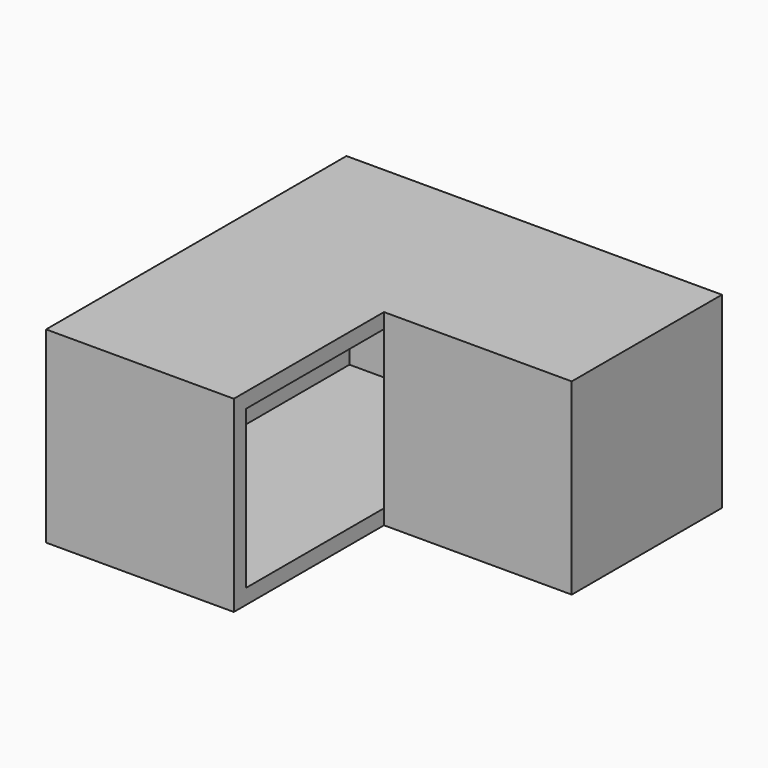
from build123d import *

# Parameters (mm, degrees)
F1_DEPTH = 150
F2_T     = -12


# Not quite as in the source:
# - a shell that OpenCascade refuses in one call is made with other operations: the cavity is built on its own and cut out


with BuildPart() as f1:
    # F0 (on Top) → F1 (new body)
    with BuildSketch(Plane.XY):
        Polygon((150, 150), (-150, 150), (-150, -150), (0, -150), (0, 0), (150, 0), align=None)
    extrude(amount=-F1_DEPTH)

    # F2: a shell. OpenCascade refuses it in one call, so the cavity is built on its own and cut out:
    # the body offset inwards by the wall thickness, plus a prism from it out through each open face.
    f2_core = offset(f1.part, amount=F2_T, kind=Kind.INTERSECTION, mode=Mode.PRIVATE)
    f2_exits = [f2_core.faces().sort_by_distance(p)[0] for p in [
        (-12, -63, -75),
    ]]
    add(f2_core, mode=Mode.SUBTRACT)
    extrude(f2_exits, amount=-F2_T, mode=Mode.SUBTRACT)


solid = f1.part
